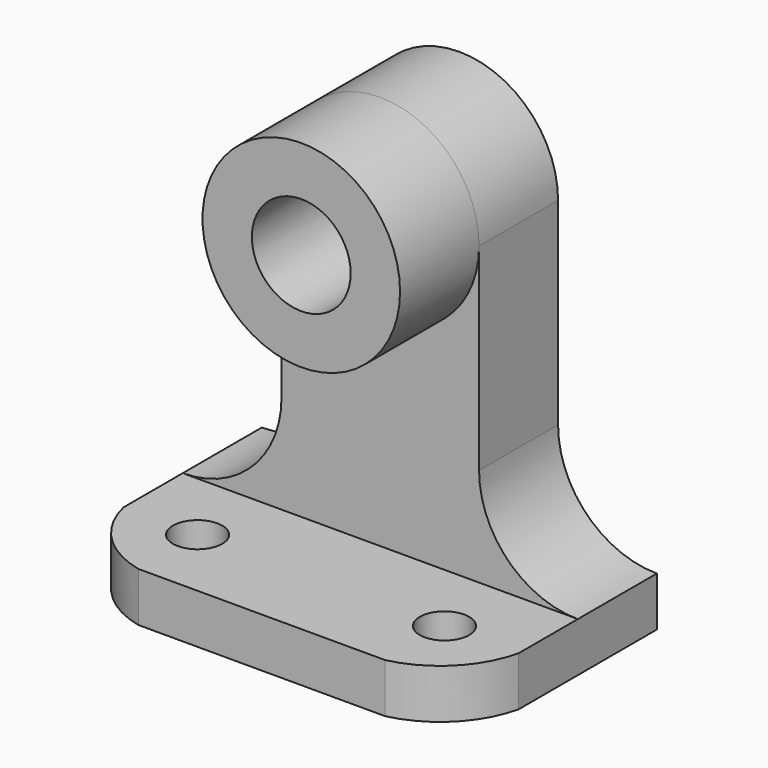
from build123d import *
from build123d import SkipClean  # not in build123d's __all__

# Parameters (mm, degrees)
F0_W      = 50.8
F0_H      = 31.75
F1_DEPTH  = 6.35
F2_R      = 3.175
F3_DEPTH  = 6.35
F4_W      = 50.8
F4_H      = 12.7
F5_DEPTH  = 57.15
F7_DEPTH  = 12.7
F8_DEPTH  = 12.7
F9_R      = 6.35
F10_DEPTH = 38.1


with BuildPart() as f1:
    # F0 (on Top) → F1 (new body)
    with BuildSketch(Plane.XY):
        with Locations((25.4, 15.875)):
            Rectangle(F0_W, F0_H)
    extrude(amount=F1_DEPTH)

    # F2 (on face) → F3 (cut)
    with BuildSketch(Plane.XY.offset(6.35)):
        with Locations((41.275, 9.525)):
            Circle(F2_R)
        with Locations((9.525, 9.525)):
            Circle(F2_R)
        with BuildLine():
            ThreePointArc((9.525, 0), (3.3956264222, 3.3956264222), (0, 9.525))
            Line((0, 9.525), (0, 0))
            Line((0, 0), (9.525, 0))
        make_face()
        with BuildLine():
            ThreePointArc((50.8, 9.525), (47.4043735778, 3.3956264222), (41.275, 0))
            Line((41.275, 0), (50.8, 0))
            Line((50.8, 0), (50.8, 9.525))
        make_face()
    extrude(amount=-F3_DEPTH, mode=Mode.SUBTRACT)

    # F4 (on face) → F5 (join)
    with BuildSketch(Plane.XY.offset(6.35)):
        with Locations((25.4, 25.4)):
            Rectangle(F4_W, F4_H)
    extrude(amount=F5_DEPTH)

    # F6 (on face) → F7 (cut)
    with BuildSketch(Plane.XZ.offset(-19.05)):
        with BuildLine():
            ThreePointArc((12.7, 44.45), (25.4, 57.15), (38.1, 44.45))
            Line((38.1, 44.45), (38.1, 19.05))
            ThreePointArc((38.1, 19.05), (41.8197438789, 10.0697438789), (50.8, 6.35))
            Line((50.8, 6.35), (50.8, 63.5))
            Line((50.8, 63.5), (0, 63.5))
            Line((0, 63.5), (0, 6.35))
            ThreePointArc((0, 6.35), (8.9802561211, 10.0697438789), (12.7, 19.05))
            Line((12.7, 19.05), (12.7, 44.45))
        make_face()
    extrude(amount=-F7_DEPTH, mode=Mode.SUBTRACT)

    # F6 (on face) → F8 (join)
    with BuildSketch(Plane.XZ.offset(-19.05)):
        with BuildLine():
            ThreePointArc((12.7, 44.45), (25.4, 31.75), (38.1, 44.45))
            ThreePointArc((38.1, 44.45), (25.4, 57.15), (12.7, 44.45))
        make_face()
    with SkipClean():  # cleaning this boolean's faces spoils the solid; the shape is the same uncleaned
        extrude(amount=F8_DEPTH)

    # F9 (on face) → F10 (cut)
    with BuildSketch(Plane.XZ.offset(-6.35)):
        with Locations((25.4, 44.45)):
            Circle(F9_R)
    with SkipClean():  # cleaning this boolean's faces spoils the solid; the shape is the same uncleaned
        extrude(amount=-F10_DEPTH, mode=Mode.SUBTRACT)


solid = f1.part
